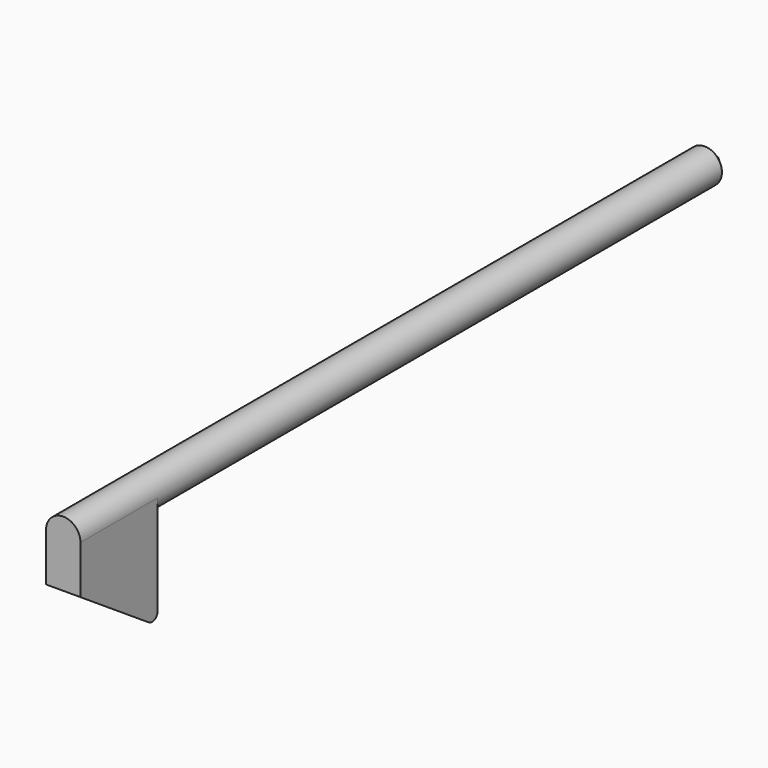
from build123d import *

# Parameters (mm, degrees)
F0_R        = 2.5
F1_DEPTH    = 105
F3_DEPTH    = 14
F4_SIZE     = 2.5
F5_T1_DEPTH = 82.5140157162
F6_R        = 1


# Not quite as in the source:
# - a fillet or chamfer that OpenCascade refuses, or shapes differently, is made with other operations: its cross-section is extruded or revolved along the edge and cut away or added


with BuildPart() as f1:
    # F0 (on Front) → F1 (new body)
    with BuildSketch(Plane.XZ):
        Circle(F0_R)
    extrude(amount=-F1_DEPTH)

    # F2 (on face) → F3 (join)
    with BuildSketch(Plane.XZ):
        with BuildLine():
            Line((-2.5, 0), (-2.5, -17))
            Line((-2.5, -17), (2.5, -17))
            Line((2.5, -17), (2.5, 0))
            ThreePointArc((2.5, 0), (0, -2.5), (-2.5, 0))
        make_face()
        with BuildLine():
            ThreePointArc((2.5, 0), (0, 2.5), (-2.5, 0))
            ThreePointArc((-2.5, 0), (0, -2.5), (2.5, 0))
        make_face()
    extrude(amount=F3_DEPTH)

    # F4
    f4_edges = [f1.edges().sort_by_distance(p)[0] for p in [
        (-2.5, 105, 0),
    ]]
    chamfer(f4_edges, length=F4_SIZE)

    # F5: chamfer of 10 x 15 on 1 edges, made by hand

    # F5_s2 → F5_t1 (cut)
    with BuildSketch(Plane.YZ.offset(-41.2570078581)):
        Polygon((-14, -7), (1, -17), (-14, -17), align=None)
    extrude(amount=F5_T1_DEPTH, mode=Mode.SUBTRACT)

    # F6
    f6_edges = [f1.edges().sort_by_distance(p)[0] for p in [
        (0, 0, -16.333333),
    ]]
    fillet(f6_edges, radius=F6_R)


solid = f1.part
